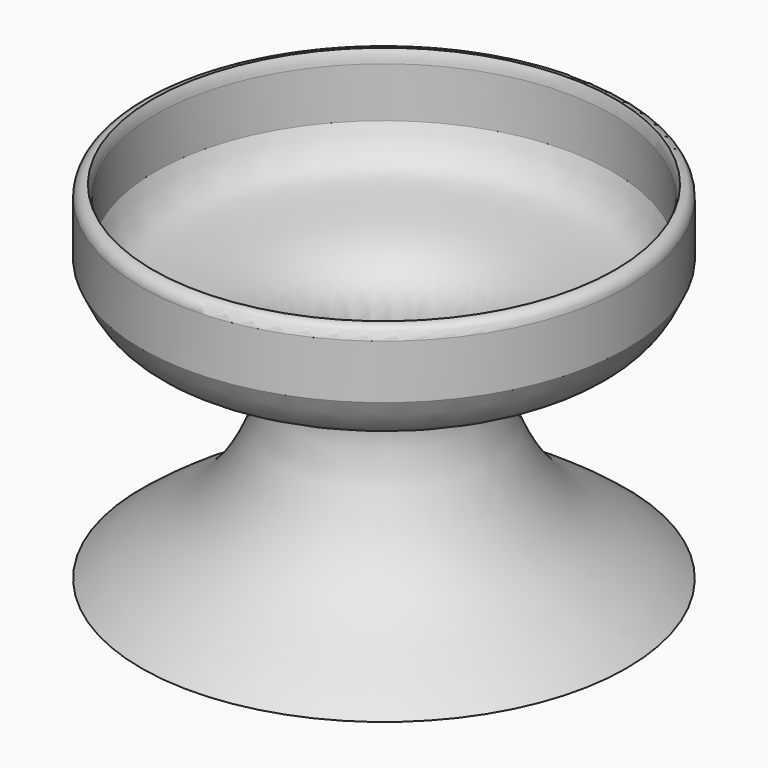
from build123d import *

# Parameters (mm, degrees)
F2_T = -2.5
F3_R = 2


# Not quite as in the source:
# - a fillet or chamfer that OpenCascade refuses, or shapes differently, is made with other operations: its cross-section is extruded or revolved along the edge and cut away or added


with BuildPart() as f1:
    # F0 (on Front) → F1 (revolve)
    with BuildSketch(Plane.XZ):
        with BuildLine():
            Line((0, 60.1978562772), (0, 0))
            Line((0, 0), (42.1288385987, 0))
            add(Edge.make_bspline(
                [(42.1288385987, 48.7960129976), (39.9398960957, 43.6724913074), (36.124754332, 39.4385747799), (11.2155060179, 39.0850801193), (23.809795732, 8.8667225507), (35.2535881514, 5.627983428), (42.1288385987, 0)],
                knots=[0, 0, 0, 0, 0.1988188163, 0.4426171309, 0.7230365515, 1, 1, 1, 1], degree=3))
            Line((42.1288385987, 48.7960129976), (42.1288385987, 60.1978562772))
            Line((42.1288385987, 60.1978562772), (0, 60.1978562772))
        make_face()
    revolve(axis=Axis((0, 0, 30.0989281386), (0, 0, 1)))

    # F2
    f2_openings = [f1.faces().sort_by_distance(p)[0] for p in [
        (0, 0, 60.197856),
    ]]
    offset(amount=F2_T, openings=f2_openings, kind=Kind.INTERSECTION)

    # F3
    f3_edges = [f1.edges().sort_by_distance(p)[0] for p in [
        (-42.128839, 0, 60.197856),
    ]]
    fillet(f3_edges, radius=F3_R)

    # F4: fillet of radius 5 on 1 edges, made by hand

    # F4_s1 → F4_t2 (revolve, cut)
    with BuildSketch(Plane.XZ):
        with BuildLine():
            ThreePointArc((40.1288385987, 60.1978562772), (39.7554414263, 59.1364407942), (39.6288385987, 58.0184068055))
            Line((39.6288385987, 58.0184068055), (39.6288385987, 60.1978562772))
            Line((39.6288385987, 60.1978562772), (40.1288385987, 60.1978562772))
        make_face()
    revolve(axis=Axis((0, 0, 60.1978562772), (0, 0, 1)), mode=Mode.SUBTRACT)


solid = f1.part
